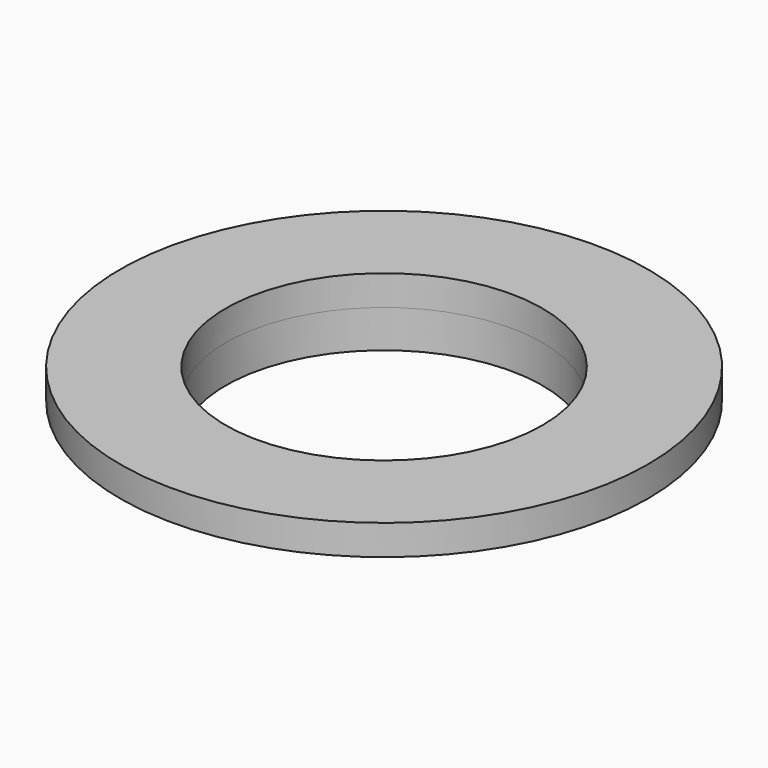
from build123d import *

# Parameters (mm, degrees)
F0_R     = 17.5
F0_R_2   = 12.5
F0_R_3   = 10.5
F1_DEPTH = 2
F2_DEPTH = 2.5


with BuildPart() as f1:
    # F0 (on Top) → F1 (new body)
    with BuildSketch(Plane.XY):
        Circle(F0_R)
        Circle(F0_R_2, mode=Mode.SUBTRACT)
        Circle(F0_R_2)
        Circle(F0_R_3, mode=Mode.SUBTRACT)
    extrude(amount=F1_DEPTH)

    # F0 (on Top) → F2 (join)
    with BuildSketch(Plane.XY):
        Circle(F0_R_2)
        Circle(F0_R_3, mode=Mode.SUBTRACT)
    extrude(amount=-F2_DEPTH)


solid = f1.part
